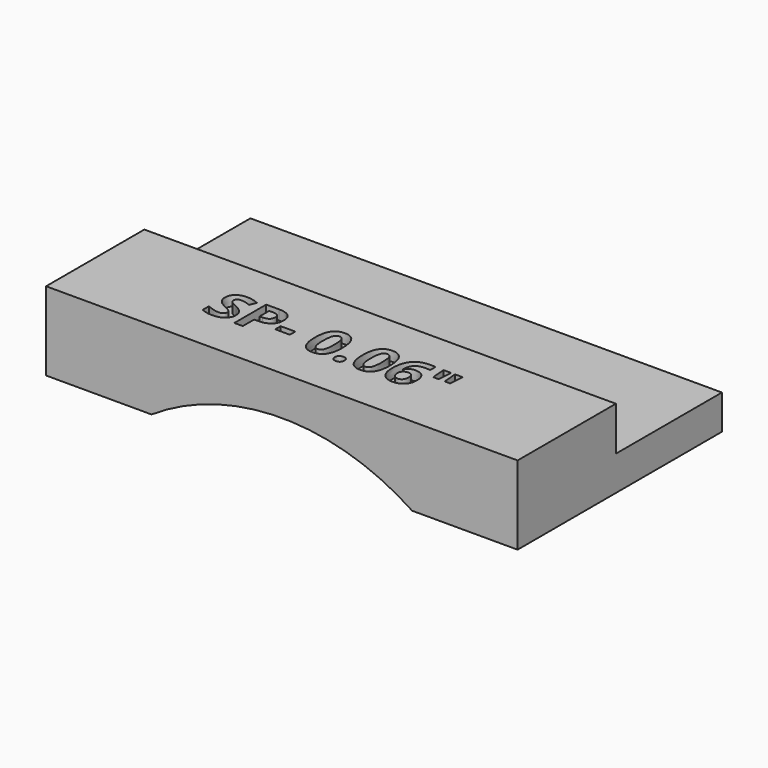
from build123d import *

# Parameters (mm, degrees)
F1_DEPTH     = 39.6875
F2_W         = 152.4
F2_H         = 25.4
F3_DEPTH     = 42.8625
F4_W         = 152.4
F4_H         = 14.224
F5_DEPTH     = 42.8498
F6_TEXT_SIZE = 18.0148498393
F7_DEPTH     = 3.175


# Not quite as in the source:
# - Text() gives the source's letters only with a copy of the font that has no kerning and outlines rounded to 1/6400 em; it was checked with that copy


with BuildPart() as f1:
    # F0 (on Front) → F1 (new body)
    with BuildSketch(Plane.XZ):
        with BuildLine():
            Line((0, 25.4), (0, 0))
            Line((0, 0), (34.0788651625, 0))
            ThreePointArc((34.0788651625, 0), (76.2, 12.7), (118.3211348375, 0))
            Line((118.3211348375, 0), (152.4, 0))
            Line((152.4, 0), (152.4, 25.4))
            Line((152.4, 25.4), (0, 25.4))
        make_face()
    extrude(amount=F1_DEPTH)

    # F2 (on face) → F3 (join)
    with BuildSketch(Plane(origin=(0, 0, 0), x_dir=(-1, 0, 0), z_dir=(0, 1, 0))):
        with Locations((-76.2, 12.7)):
            Rectangle(F2_W, F2_H)
    extrude(amount=F3_DEPTH)

    # F4 (on face) → F5 (cut)
    with BuildSketch(Plane(origin=(0, 42.8625, 0), x_dir=(-1, 0, 0), z_dir=(0, 1, 0))):
        with Locations((-76.2, 18.288)):
            Rectangle(F4_W, F4_H)
    extrude(amount=-F5_DEPTH, mode=Mode.SUBTRACT)

    # F6 (on face) → F7 (cut)
    with BuildSketch(Plane.XY.offset(25.4)):
        with Locations((38.1, -25.6706918843)):
            Text('SP- 0.06"', F6_TEXT_SIZE, font='Open Sans', font_style=FontStyle.BOLD, text_align=(TextAlign.LEFT, TextAlign.BOTTOM))
    extrude(amount=-F7_DEPTH, mode=Mode.SUBTRACT)


solid = f1.part
